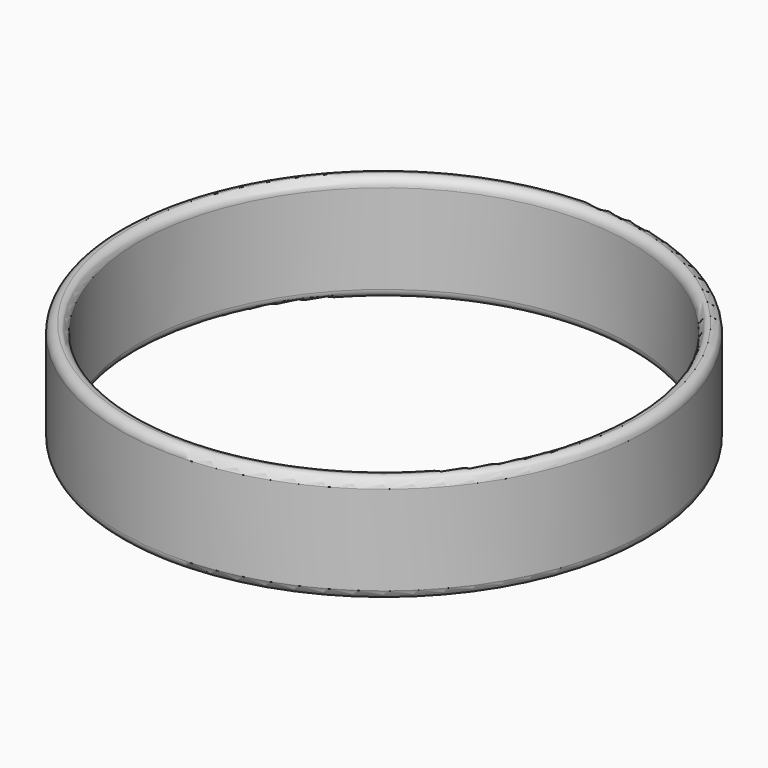
from build123d import *

# Parameters (mm, degrees)
F0_R     = 29.5
F0_R_2   = 27.5
F1_DEPTH = 12
F2_R     = 0.99999


# Not quite as in the source:
# - a fillet or chamfer is up to 0.001 mm smaller than in the source, because OpenCascade refuses the exact size


with BuildPart() as f1:
    # F0 (on Top) → F1 (new body)
    with BuildSketch(Plane.XY):
        Circle(F0_R)
        Circle(F0_R_2, mode=Mode.SUBTRACT)
    extrude(amount=F1_DEPTH)

    # F2 (radius 1 in the source; OpenCascade refuses exactly that, so slightly less here)
    f2_edges = [f1.edges().sort_by_distance(p)[0] for p in [
        (-29.5, 0, 12),
        (-27.5, 0, 12),
        (-29.5, 0, 0),
        (-27.5, 0, 0),
    ]]
    fillet(f2_edges, radius=F2_R)


solid = f1.part
